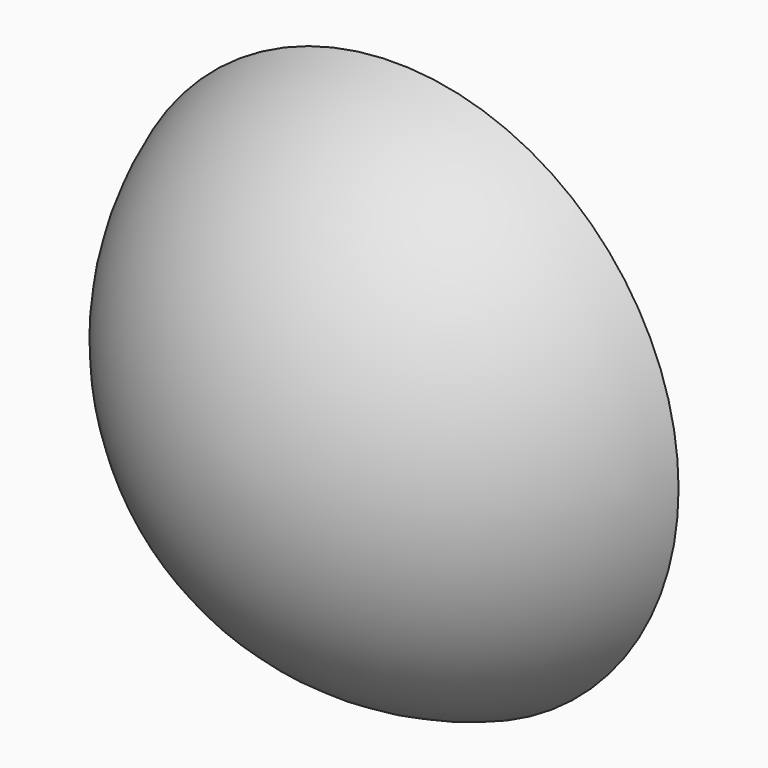
from build123d import *


# Not quite as in the source:
# - the program builds the solid bodies; features that only make, move or delete a surface that nothing else refers to are left out


with BuildPart() as f2:
    # F0 (on Top) → F2 (revolve)
    with BuildSketch(Plane.XY):
        with BuildLine():
            Line((12500, 0), (0, 0))
            Line((0, 0), (0, -8500))
            ThreePointArc((0, -8500), (7558.1082289155, -6173.6885719345), (12500, 0))
        make_face()
        with BuildLine():
            ThreePointArc((12500, 0), (7558.1082289155, -6173.6885719345), (0, -8500))
            Line((0, -8500), (0, -9000))
            ThreePointArc((0, -9000), (7701.4609003747, -6515.9179171871), (12500, 0))
        make_face()
    revolve(axis=Axis((0, -4250, 0), (0, -1, 0)))


solid = f2.part
